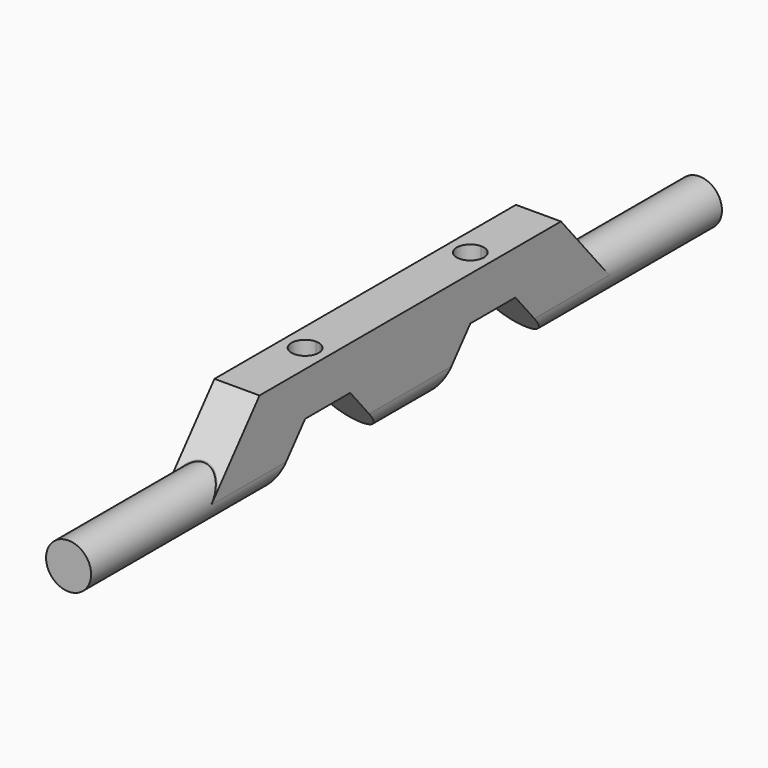
from build123d import *

# Parameters (mm, degrees)
F0_R      = 2.5
F1_DEPTH  = 85
F3_DEPTH  = 2.5
F5_DEPTH  = 25
F8_DEPTH  = 25
F9_DEPTH  = 25
F11_DEPTH = 25
F14_DEPTH = 102
F16_REACH = 96.5783545855
F18_REACH = 97.7333268634
F19_DEPTH = 1


with BuildPart() as f1:
    # F0 (on Front) → F1 (new body)
    with BuildSketch(Plane.XZ):
        Circle(F0_R)
    extrude(amount=F1_DEPTH)

    # F2 (on Right) → F3 (join, symmetric)
    with BuildSketch(Plane.YZ):
        Polygon((-69, 0), (-16, 0), (-22.4278760969, 7.6604444312), (-62.5721239031, 7.6604444312), align=None)
    extrude(amount=F3_DEPTH, both=True)

    # F4 (on face) → F5 (cut)
    with BuildSketch(Plane(origin=(-2.5, 0, 0), x_dir=(0, -1, 0), z_dir=(-1, 0, 0))):
        Polygon((56.5, 3), (53.5, 3), (50.5, 3), (44.1691353238, -4.5448307221), (62.8308646762, -4.5448307221), align=None)
        Polygon((40.8308646762, -4.5448307221), (34.5, 3), (31.5, 3), (28.5, 3), (22.1691353238, -4.5448307221), align=None)
    extrude(amount=-F5_DEPTH, mode=Mode.SUBTRACT)

    # F7 (on face) → F8 (cut)
    with BuildSketch(Plane(origin=(-2.5, 0, 0), x_dir=(0, -1, 0), z_dir=(-1, 0, 0))):
        Polygon((19.9172031134, 7.5), (22.2932472338, 7.5), (22.4278760969, 7.6604444312), (62.5721239031, 7.6604444312), (62.7067527662, 7.5), (66.5233954787, 7.5), (66.5233954787, 10.3880958632), (19.9172031134, 10.3880958632), align=None)
    extrude(amount=-F8_DEPTH, mode=Mode.SUBTRACT)

    # F6 (on face) → F9 (cut)
    with BuildSketch(Plane(origin=(0, 0, 3), x_dir=(1, 0, 0), z_dir=(0, 0, -1))):
        with BuildLine():
            ThreePointArc((1.45, 53.5), (1.0253048327, 54.5253048327), (0, 54.95))
            Line((0, 54.95), (0, 52.05))
            ThreePointArc((0, 52.05), (1.0253048327, 52.4746951673), (1.45, 53.5))
        make_face()
        with BuildLine():
            Line((0, 52.05), (0, 54.95))
            ThreePointArc((0, 54.95), (-1.45, 53.5), (0, 52.05))
        make_face()
    extrude(amount=-F9_DEPTH, mode=Mode.SUBTRACT)

    # F10 (on face) → F11 (cut)
    with BuildSketch(Plane(origin=(0, 0, 3), x_dir=(1, 0, 0), z_dir=(0, 0, -1))):
        with BuildLine():
            ThreePointArc((1.45, 31.5), (1.0253048327, 32.5253048327), (0, 32.95))
            Line((0, 32.95), (0, 30.05))
            ThreePointArc((0, 30.05), (1.0253048327, 30.4746951673), (1.45, 31.5))
        make_face()
        with BuildLine():
            Line((0, 30.05), (0, 32.95))
            ThreePointArc((0, 32.95), (-1.45, 31.5), (0, 30.05))
        make_face()
    extrude(amount=-F11_DEPTH, mode=Mode.SUBTRACT)

    # F13 (on face) → F14 (cut)
    with BuildSketch(Plane.XZ.offset(85)):
        with BuildLine():
            ThreePointArc((2.4, 0), (0, -2.4), (-2.4, 0))
            Line((-2.4, 0), (-2.4, 9.7710704431))
            Line((-2.4, 9.7710704431), (-6.1972029507, 9.7710704431))
            Line((-6.1972029507, 9.7710704431), (-6.1972029507, -5.7614380494))
            Line((-6.1972029507, -5.7614380494), (5.5722752586, -5.7614380494))
            Line((5.5722752586, -5.7614380494), (5.5722752586, 8.8547384366))
            Line((5.5722752586, 8.8547384366), (2.4, 9.1607915238))
            Line((2.4, 9.1607915238), (2.4, 0))
        make_face()
    extrude(amount=-F14_DEPTH, mode=Mode.SUBTRACT)

    f16_end = Plane(origin=(0, -64.9529870595, 4.8230422111), x_dir=(0, -0.6427876097, -0.7660444431), z_dir=(0, -0.7660444431, 0.6427876097))
    # F15 (on face) → F16 (cut, up to a plane its end follows)
    with BuildSketch(Plane.XZ.offset(85)):
        with BuildLine():
            ThreePointArc((-2.4, 0), (0, 2.4), (2.4, 0))
            Line((2.4, 0), (4.8319334164, 0))
            Line((4.8319334164, 0), (4.1808704846, 8.0774491653))
            Line((4.1808704846, 8.0774491653), (-2.9383567162, 8.0774491653))
            Line((-2.9383567162, 8.0774491653), (-3.4620375372, 0))
            Line((-3.4620375372, 0), (-2.4, 0))
        make_face()
    f16_long = extrude(amount=-F16_REACH, mode=Mode.PRIVATE)
    add(split(f16_long, bisect_by=f16_end, keep=Keep.TOP, mode=Mode.PRIVATE), mode=Mode.SUBTRACT)

    f18_end = Plane(origin=(0, -20.0470129405, 4.8230422111), x_dir=(0, -0.6427876097, 0.7660444431), z_dir=(0, 0.7660444431, 0.6427876097))
    # F17 (on face) → F18 (cut, up to a plane its end follows)
    with BuildSketch(Plane(origin=(0, 0, 0), x_dir=(-1, 0, 0), z_dir=(0, 1, 0))):
        with BuildLine():
            ThreePointArc((-2.4, 0), (0, 2.4), (2.4, 0))
            Line((2.4, 0), (3.9089121856, 0))
            Line((3.9089121856, 0), (4.3247276917, 8.6870230734))
            Line((4.3247276917, 8.6870230734), (-4.9837511033, 8.3660408854))
            Line((-4.9837511033, 8.3660408854), (-3.4170385916, 0))
            Line((-3.4170385916, 0), (-2.4, 0))
        make_face()
    f18_long = extrude(amount=-F18_REACH, mode=Mode.PRIVATE)
    add(split(f18_long, bisect_by=f18_end, keep=Keep.TOP, mode=Mode.PRIVATE), mode=Mode.SUBTRACT)

    # F19 (cut): a face of the model
    f19_faces = [f1.faces().sort_by_distance(p)[0] for p in [
        (0, 0, 0),
    ]]
    extrude(f19_faces, amount=-F19_DEPTH, mode=Mode.SUBTRACT)


solid = f1.part
